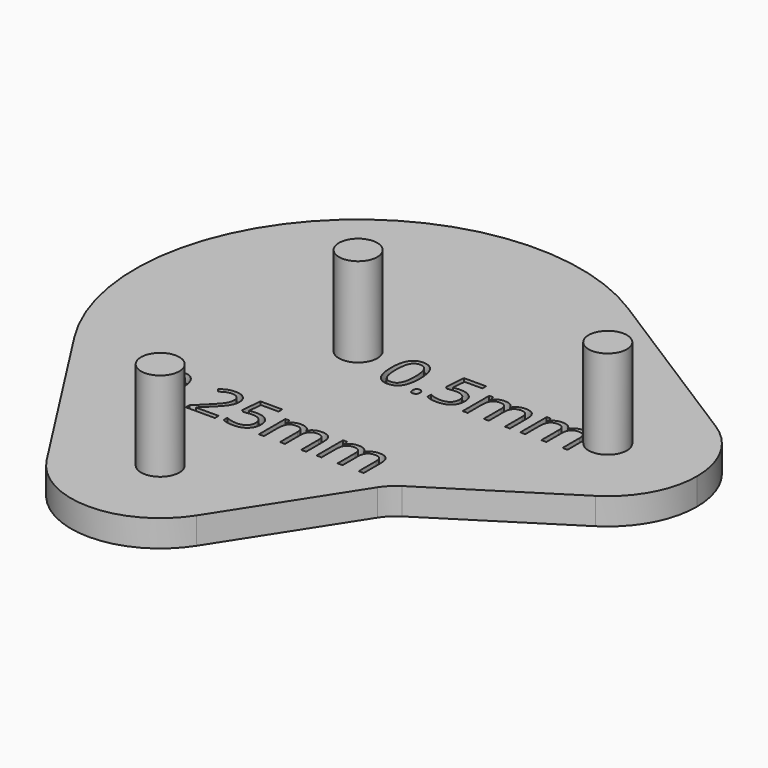
from build123d import *

# Parameters (mm, degrees)
F1_DEPTH     = 3
F3_R         = 2.15
F4_DEPTH     = 10
F5_TEXT_SIZE = 6.9444444444
F6_DEPTH     = 1


# Not quite as in the source:
# - a feature names something its author has since deleted; it is built from what else it names
# - Text() gives the source's letters only with a copy of the font that has no kerning and outlines rounded to 1/6400 em; it was checked with that copy


with BuildPart() as f1:
    # F0 (on Top) → F1 (new body)
    with BuildSketch(Plane.XY):
        with BuildLine():
            ThreePointArc((-10.3719737087, 8.8661928132), (-14.37053367, 15.7972646819), (-20.3541165658, 21.1099828885))
            ThreePointArc((-20.3541165658, 21.1099828885), (-51.4751822329, 17.6269856335), (-54.7799229199, -13.5135135135))
            ThreePointArc((-54.7799229199, -13.5135135135), (-49.5327960665, -19.3857631391), (-42.7193202097, -23.3344594595))
            ThreePointArc((-42.7193202097, -23.3344594595), (-39.0311290146, -19.2601411848), (-33.7469737087, -17.75))
            Line((-33.7469737087, -17.75), (-33.7469737087, -2.25))
            ThreePointArc((-33.7469737087, -2.25), (-35.3379639664, 1.5909902577), (-31.4969737087, 0))
            Line((-31.4969737087, 0), (-15.7469737087, 0))
            ThreePointArc((-15.7469737087, 0), (-14.2982893969, 5.1841103383), (-10.3719737087, 8.8661928132))
        make_face()
        with BuildLine():
            Line((-0.3898308516, 8.4439931554), (-20.3541165658, 21.1099828885))
            ThreePointArc((-20.3541165658, 21.1099828885), (-14.37053367, 15.7972646819), (-10.3719737087, 8.8661928132))
            ThreePointArc((-10.3719737087, 8.8661928132), (-5.3243965813, 9.991067439), (-0.3898308516, 8.4439931554))
        make_face()
        with BuildLine():
            ThreePointArc((-42.7193202097, -23.3344594595), (-49.5327960665, -19.3857631391), (-54.7799229199, -13.5135135135))
            Line((-54.7799229199, -13.5135135135), (-42.1601533932, -33.1554054054))
            ThreePointArc((-42.1601533932, -33.1554054054), (-43.7308043866, -28.3184408455), (-42.7193202097, -23.3344594595))
        make_face()
        with BuildLine():
            ThreePointArc((-0.3898308516, 8.4439931554), (-5.3243965813, 9.991067439), (-10.3719737087, 8.8661928132))
            ThreePointArc((-10.3719737087, 8.8661928132), (-9.1565792426, 4.5069390943), (-8.7469737087, 0))
            ThreePointArc((-8.7469737087, 0), (-9.1565792426, -4.5069390943), (-10.3719737087, -8.8661928132))
            ThreePointArc((-10.3719737087, -8.8661928132), (-5.3243965813, -9.991067439), (-0.3898308516, -8.4439931554))
            ThreePointArc((-0.3898308516, -8.4439931554), (3.0157721101, -4.8181205583), (4.2530262913, 0))
            ThreePointArc((4.2530262913, 0), (3.0157721101, 4.8181205583), (-0.3898308516, 8.4439931554))
        make_face()
        with BuildLine():
            ThreePointArc((-3.4969737087, 0), (-5.7469737087, -2.25), (-7.9969737087, 0))
            ThreePointArc((-7.9969737087, 0), (-5.7469737087, 2.25), (-3.4969737087, 0))
        make_face(mode=Mode.SUBTRACT)
        with BuildLine():
            ThreePointArc((-33.7469737087, -25), (-38.3097860823, -24.580088349), (-42.7193202097, -23.3344594595))
            ThreePointArc((-42.7193202097, -23.3344594595), (-43.7308043866, -28.3184408455), (-42.1601533932, -33.1554054054))
            ThreePointArc((-42.1601533932, -33.1554054054), (-33.7469737087, -37.75), (-25.3337940242, -33.1554054054))
            ThreePointArc((-25.3337940242, -33.1554054054), (-24.1518760843, -30.5667537304), (-23.7469737087, -27.75))
            ThreePointArc((-23.7469737087, -27.75), (-24.0072749195, -25.4832253101), (-24.7746272077, -23.3344594595))
            ThreePointArc((-24.7746272077, -23.3344594595), (-29.1841613351, -24.580088349), (-33.7469737087, -25))
        make_face()
        with BuildLine():
            ThreePointArc((-31.4969737087, -27.75), (-35.3379639664, -29.3409902577), (-33.7469737087, -25.5))
            ThreePointArc((-33.7469737087, -25.5), (-32.155983451, -26.1590097423), (-31.4969737087, -27.75))
        make_face(mode=Mode.SUBTRACT)
        with BuildLine():
            ThreePointArc((-23.7469737087, -27.75), (-24.1518760843, -30.5667537304), (-25.3337940242, -33.1554054054))
            Line((-25.3337940242, -33.1554054054), (-16.2923281862, -19.0829222148))
            ThreePointArc((-16.2923281862, -19.0829222148), (-15.6111354707, -18.2399832127), (-14.7643097726, -17.5636283398))
            Line((-14.7643097726, -17.5636283398), (-0.3898308516, -8.4439931554))
            ThreePointArc((-0.3898308516, -8.4439931554), (-5.3243965813, -9.991067439), (-10.3719737087, -8.8661928132))
            ThreePointArc((-10.3719737087, -8.8661928132), (-16.0291749924, -17.6374490403), (-24.7746272077, -23.3344594595))
            ThreePointArc((-24.7746272077, -23.3344594595), (-24.0072749195, -25.4832253101), (-23.7469737087, -27.75))
        make_face()
        with BuildLine():
            ThreePointArc((-10.3719737087, -8.8661928132), (-9.1565792426, -4.5069390943), (-8.7469737087, 0))
            Line((-8.7469737087, 0), (-15.7469737087, 0))
            ThreePointArc((-15.7469737087, 0), (-14.2982893969, -5.1841103383), (-10.3719737087, -8.8661928132))
        make_face()
        with BuildLine():
            ThreePointArc((-31.4969737087, -27.75), (-32.155983451, -26.1590097423), (-33.7469737087, -25.5))
            ThreePointArc((-33.7469737087, -25.5), (-35.3379639664, -29.3409902577), (-31.4969737087, -27.75))
        make_face()
        with BuildLine():
            ThreePointArc((-33.7469737087, -2.25), (-32.155983451, -1.5909902577), (-31.4969737087, 0))
            Line((-31.4969737087, 0), (-33.7469737087, 0))
            Line((-33.7469737087, 0), (-33.7469737087, -2.25))
        make_face()
        with BuildLine():
            Line((-33.7469737087, 0), (-31.4969737087, 0))
            ThreePointArc((-31.4969737087, 0), (-35.3379639664, 1.5909902577), (-33.7469737087, -2.25))
            Line((-33.7469737087, -2.25), (-33.7469737087, 0))
        make_face()
        with BuildLine():
            ThreePointArc((-3.4969737087, 0), (-5.7469737087, 2.25), (-7.9969737087, 0))
            ThreePointArc((-7.9969737087, 0), (-5.7469737087, -2.25), (-3.4969737087, 0))
        make_face()
        with BuildLine():
            Line((-33.7469737087, -17.75), (-33.7469737087, -25))
            ThreePointArc((-33.7469737087, -25), (-29.1841613351, -24.580088349), (-24.7746272077, -23.3344594595))
            ThreePointArc((-24.7746272077, -23.3344594595), (-28.4628184028, -19.2601411848), (-33.7469737087, -17.75))
        make_face()
        with BuildLine():
            ThreePointArc((-33.7469737087, -17.75), (-39.0311290146, -19.2601411848), (-42.7193202097, -23.3344594595))
            ThreePointArc((-42.7193202097, -23.3344594595), (-38.3097860823, -24.580088349), (-33.7469737087, -25))
            Line((-33.7469737087, -25), (-33.7469737087, -17.75))
        make_face()
        with BuildLine():
            ThreePointArc((-8.7469737087, 0), (-9.1565792426, 4.5069390943), (-10.3719737087, 8.8661928132))
            ThreePointArc((-10.3719737087, 8.8661928132), (-14.2982893969, 5.1841103383), (-15.7469737087, 0))
            Line((-15.7469737087, 0), (-8.7469737087, 0))
        make_face()
        with BuildLine():
            ThreePointArc((-10.3719737087, -8.8661928132), (-14.2982893969, -5.1841103383), (-15.7469737087, 0))
            Line((-15.7469737087, 0), (-31.4969737087, 0))
            ThreePointArc((-31.4969737087, 0), (-32.155983451, -1.5909902577), (-33.7469737087, -2.25))
            Line((-33.7469737087, -2.25), (-33.7469737087, -17.75))
            ThreePointArc((-33.7469737087, -17.75), (-28.4628184028, -19.2601411848), (-24.7746272077, -23.3344594595))
            ThreePointArc((-24.7746272077, -23.3344594595), (-16.0291749924, -17.6374490403), (-10.3719737087, -8.8661928132))
        make_face()
    extrude(amount=F1_DEPTH)

    # F3 (on face) → F4 (join)
    with BuildSketch(Plane.XY.offset(3)):
        with Locations((-33.7469737087, -27.75)):
            Circle(F3_R)
        with Locations((-5.7469737087, 0)):
            Circle(F3_R)
        with Locations((-33.7469737087, 0)):
            Circle(F3_R)
    extrude(amount=F4_DEPTH)

    # F5 (on face) → F6 (cut)
    with BuildSketch(Plane.XY.offset(3)):
        with Locations((-29.890612036, -3.1479658636)):
            Text('0.5mm', F5_TEXT_SIZE, font='Open Sans', text_align=(TextAlign.LEFT, TextAlign.BOTTOM))
        with Locations((-45.0479153571, -17.7304829657)):
            Text('0.25mm', F5_TEXT_SIZE, font='Open Sans', text_align=(TextAlign.LEFT, TextAlign.BOTTOM))
    extrude(amount=-F6_DEPTH, mode=Mode.SUBTRACT)


solid = f1.part
